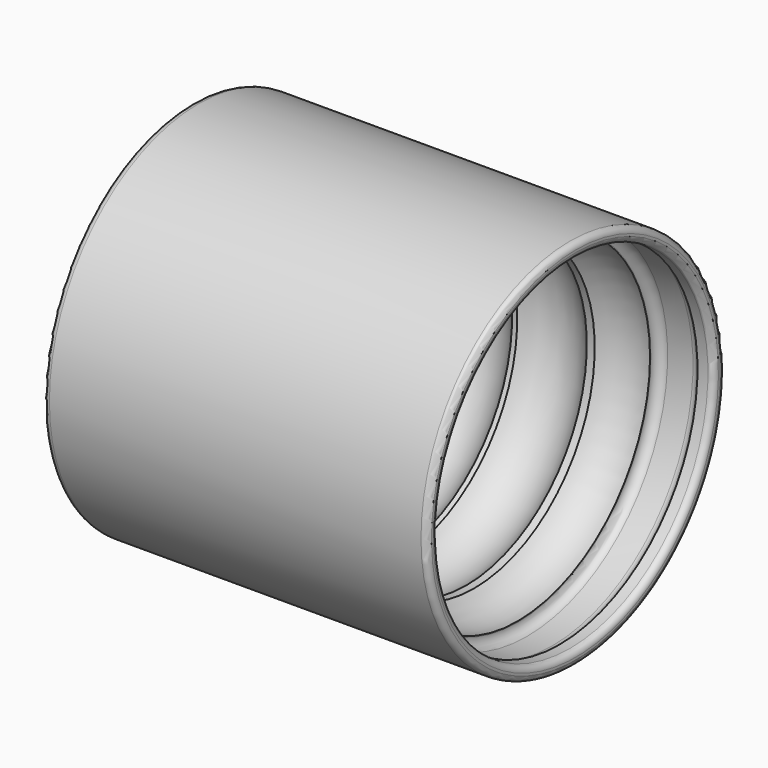
from build123d import *

# Parameters (mm, degrees)
F2_R = 0.5
F4_R = 1.25
F5_R = 1.5


# Not quite as in the source:
# - a fillet or chamfer that OpenCascade refuses, or shapes differently, is made with other operations: its cross-section is extruded or revolved along the edge and cut away or added


with BuildPart() as f1:
    # F0 (on Front) → F1 (revolve)
    with BuildSketch(Plane.XZ):
        with BuildLine():
            Line((82.5, 37), (82.5, 40))
            Line((82.5, 40), (0, 40))
            Line((0, 40), (0, 31))
            Line((0, 31), (5, 31))
            Line((5, 31), (5, 34.8))
            Line((5, 34.8), (10, 34.8))
            Line((10, 34.8), (10, 31))
            Line((10, 31), (11.4, 31))
            ThreePointArc((11.4, 31), (19.0365134749, 35.6643650208), (27.3484099858, 32.35))
            Line((27.3484099858, 32.35), (28.4484099858, 32.35))
            ThreePointArc((28.4484099858, 32.35), (35.6899882075, 35.7), (42.9315664293, 32.35))
            Line((42.9315664293, 32.35), (44.0315664293, 32.35))
            ThreePointArc((44.0315664293, 32.35), (51.5, 35.7), (58.9684335707, 32.35))
            Line((58.9684335707, 32.35), (60.6684335707, 32.35))
            ThreePointArc((60.6684335707, 32.35), (64.9158653321, 35.1670558963), (70, 35.5249038647))
            Line((70, 35.5249038647), (70, 37.75))
            Line((70, 37.75), (79, 37.75))
            Line((79, 37.75), (79, 37))
            Line((79, 37), (82.5, 37))
        make_face()
    revolve(axis=Axis((2.4749229779, 0, 0), (1, 0, 0)))

    # F2
    f2_edges = [f1.edges().sort_by_distance(p)[0] for p in [
        (5, 0, -34.8),
        (10, 0, -34.8),
    ]]
    fillet(f2_edges, radius=F2_R)

    # F3: fillet of radius 2 on 2 edges, made by hand

    # F3_s1 → F3_t2 (revolve)
    with BuildSketch(Plane.XZ):
        with BuildLine():
            ThreePointArc((72, 37.75), (70.5857864376, 37.1642135624), (70, 35.75))
            Line((70, 35.75), (70, 37.75))
            Line((70, 37.75), (72, 37.75))
        make_face()
    revolve(axis=Axis((70, 0, 0), (1, 0, 0)))

    # F3_s3 → F3_t4 (revolve)
    with BuildSketch(Plane.XZ):
        with BuildLine():
            ThreePointArc((79, 37), (78.3047759042, 37.5527756377), (77.4387505004, 37.75))
            Line((77.4387505004, 37.75), (79, 37.75))
            Line((79, 37.75), (79, 37))
        make_face()
    revolve(axis=Axis((79, 0, 0), (1, 0, 0)))

    # F4
    f4_edges = [f1.edges().sort_by_distance(p)[0] for p in [
        (82.5, 0, -40),
        (82.5, 0, -37),
    ]]
    fillet(f4_edges, radius=F4_R)

    # F5
    f5_edges = [f1.edges().sort_by_distance(p)[0] for p in [
        (0, 0, -40),
    ]]
    fillet(f5_edges, radius=F5_R)


solid = f1.part
